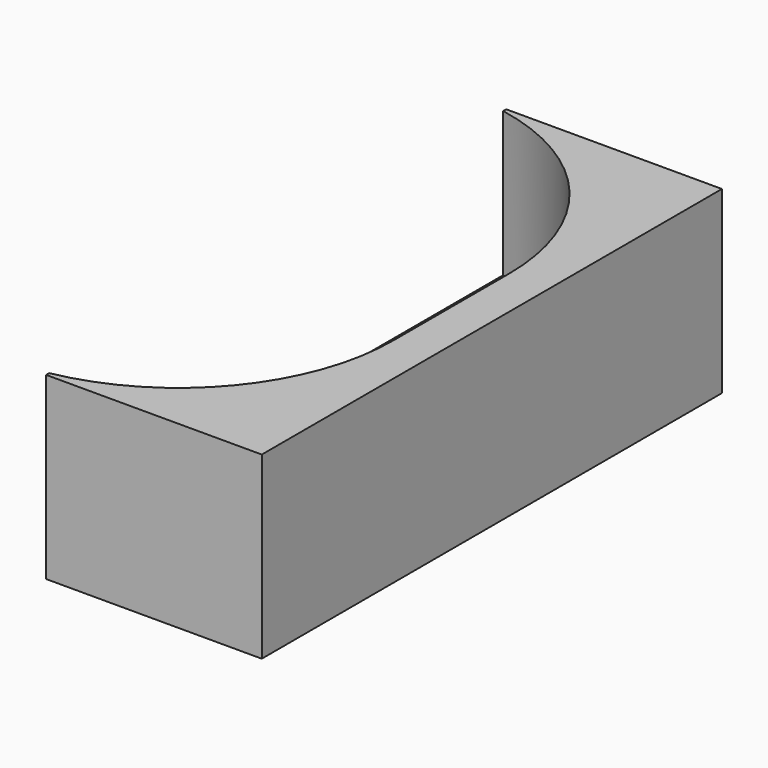
from build123d import *

# Parameters (mm, degrees)
F1_DEPTH    = 80
F2_T1_DEPTH = 140
F2_T3_DEPTH = 85
F2_T6_ANGLE = 90
F2_T8_ANGLE = 90
F3_W        = 30
F3_H        = 80
F4_DEPTH    = 25


# Not quite as in the source:
# - a fillet or chamfer that OpenCascade refuses, or shapes differently, is made with other operations: its cross-section is extruded or revolved along the edge and cut away or added


with BuildPart() as f1:
    # F0 (on Front) → F1 (new body)
    with BuildSketch(Plane.XZ):
        with BuildLine():
            Line((85, 129.9038105677), (75, 129.9038105677))
            Line((75, 129.9038105677), (0, 0))
            Line((0, 0), (16.9389196682, 0))
            Line((16.9389196682, 0), (16.9389196682, 4.9038105677))
            Line((16.9389196682, 4.9038105677), (34.5854811567, 4.9038105677))
            Line((34.5854811567, 4.9038105677), (34.5854811567, 6.5063509461))
            ThreePointArc((34.5854811567, 6.5063509461), (36.2891898423, 19.4473032012), (41.2842109675, 31.5063509461))
            Line((41.2842109675, 31.5063509461), (86.5319459163, 109.8777268049))
            ThreePointArc((86.5319459163, 109.8777268049), (117.3568969946, 96.1773012088), (130, 64.9038105677))
            ThreePointArc((130, 64.9038105677), (127.4711560413, 41.3606586971), (120, 18.8916382651))
            Line((120, 18.8916382651), (120, 4.9038105677))
            Line((120, 4.9038105677), (135, 4.9038105677))
            Line((135, 4.9038105677), (135, -0.0961894323))
            Line((135, -0.0961894323), (150, -0.0961894323))
            Line((150, -0.0961894323), (150, 64.9038105677))
            ThreePointArc((150, 64.9038105677), (130.9619407771, 110.8657513448), (85, 129.9038105677))
        make_face()
    extrude(amount=F1_DEPTH)

    # F2: fillet of radius 30 on 2 edges, made by hand

    # F2_s2 → F2_t1 (cut)
    with BuildSketch(Plane.XY.offset(-75.0961894323)):
        with BuildLine():
            ThreePointArc((150, -50), (141.2132034356, -71.2132034356), (120, -80))
            Line((120, -80), (150, -80))
            Line((150, -80), (150, -50))
        make_face()
        with BuildLine():
            ThreePointArc((150, -30), (141.2132034356, -8.7867965644), (120, 0))
            Line((120, 0), (150, 0))
            Line((150, 0), (150, -30))
        make_face()
    extrude(amount=F2_T1_DEPTH, mode=Mode.SUBTRACT)

    # F2_s4 → F2_t3 (cut)
    with BuildSketch(Plane.YZ):
        with BuildLine():
            ThreePointArc((-50, 129.9038105677), (-71.2132034356, 121.1170140033), (-80, 99.9038105677))
            Line((-80, 99.9038105677), (-80, 129.9038105677))
            Line((-80, 129.9038105677), (-50, 129.9038105677))
        make_face()
        with BuildLine():
            ThreePointArc((-30, 129.9038105677), (-8.7867965644, 121.1170140033), (0, 99.9038105677))
            Line((0, 99.9038105677), (0, 129.9038105677))
            Line((0, 129.9038105677), (-30, 129.9038105677))
        make_face()
    extrude(amount=F2_T3_DEPTH, mode=Mode.SUBTRACT)

    # F2_s5 → F2_t6 (revolve, cut)
    with BuildSketch(Plane.XY.offset(64.9038105677)):
        with BuildLine():
            ThreePointArc((150, -30), (141.2132034356, -8.7867965644), (120, 0))
            Line((120, 0), (150, 0))
            Line((150, 0), (150, -30))
        make_face()
    revolve(axis=Axis((85, 0, 64.9038105677), (0, -1, 0)), revolution_arc=F2_T6_ANGLE, mode=Mode.SUBTRACT)

    # F2_s7 → F2_t8 (revolve, cut)
    with BuildSketch(Plane.XY.offset(64.9038105677)):
        with BuildLine():
            ThreePointArc((150, -50), (141.2132034356, -71.2132034356), (120, -80))
            Line((120, -80), (150, -80))
            Line((150, -80), (150, -50))
        make_face()
    revolve(axis=Axis((85, -80, 64.9038105677), (0, -1, 0)), revolution_arc=F2_T8_ANGLE, mode=Mode.SUBTRACT)


with BuildPart() as f4:
    # F3 (on Top) → F4 (new body)
    with BuildSketch(Plane.XY):
        with Locations((140.605225563, -40)):
            Rectangle(F3_W, F3_H)
    extrude(amount=F4_DEPTH)

    # F5: cut F1
    add(f1.part, mode=Mode.SUBTRACT)


solid = f4.part
